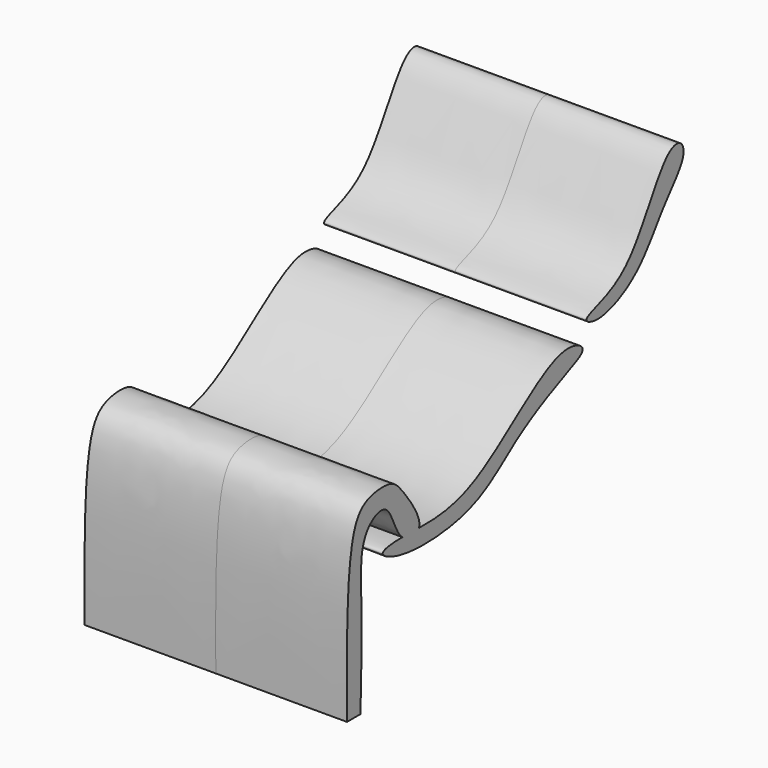
from build123d import *

# Parameters (mm, degrees)
F1_DEPTH = 63.5


with BuildPart() as f1:
    # F0 (on Right) → F1 (new body, symmetric)
    with BuildSketch(Plane.YZ):
        with BuildLine():
            add(Edge.make_bspline(
                [(-143.2403773069, -104.3510586023), (-142.7562305545, -88.6156108717), (-141.8814850282, -60.1848867372), (-144.5745803778, -27.8573641543), (-124.9688455585, -18.2280926487), (-122.6595201023, -35.2702398919), (-117.8873968399, -39.2565765031)],
                knots=[0, 0, 0, 0, 0.144009507, 0.260189796, 0.3348491633, 0.4268115335, 0.4268115335, 0.4268115335, 0.4268115335], degree=3))
            add(Edge.make_bspline(
                [(-117.8873968399, -39.2565765031), (-114.7446942469, -39.2553643323), (-111.3888290008, -39.3884462115), (-107.8556342883, -39.4389297117)],
                knots=[0, 0, 0, 0, 0.037982426, 0.037982426, 0.037982426, 0.037982426], degree=3))
            add(Edge.make_bspline(
                [(-107.8556342883, -39.4389297117), (-106.063178392, -35.3439779029), (-118.296132153, -18.3972227692), (-124.2406833684, -12.5728886668), (-138.4186777931, -13.1151114694), (-151.9247554576, -23.7874876821), (-151.6138692557, -70.8019272139), (-151.3920426369, -104.3510586023)],
                knots=[0.4939256363, 0.4939256363, 0.4939256363, 0.4939256363, 0.5938790041, 0.6592806539, 0.732580388, 0.809166244, 1, 1, 1, 1], degree=3))
            add(Edge.make_bspline(
                [(-151.3920426369, -104.3510586023), (-148.6748208602, -104.3510586023), (-145.9575990836, -104.3510586023), (-143.2403773069, -104.3510586023)],
                knots=[0, 0, 0, 0, 8.1516653299, 8.1516653299, 8.1516653299, 8.1516653299], degree=3))
        make_face()
        with BuildLine():
            add(Edge.make_bspline(
                [(-117.8873968399, -39.2565765031), (-114.4047030965, -42.165803447), (-109.0591862239, -42.1885020642), (-107.8556342883, -39.4389297117)],
                knots=[0.4268115335, 0.4268115335, 0.4268115335, 0.4268115335, 0.4939256363, 0.4939256363, 0.4939256363, 0.4939256363], degree=3))
            add(Edge.make_bspline(
                [(-107.8556342883, -39.4389297117), (-98.5103778433, -39.5724579472), (-69.6510901191, -38.3611280454), (-27.0967446465, 6.9957296893), (-3.7261879502, -3.5535051081), (-20.8971455397, -10.6520081189), (-49.7921916514, -24.3192169011), (-72.345637494, -47.096617427), (-117.0643868308, -49.4816010583), (-134.6082046549, -40.2850495858), (-124.0601600445, -39.2589573977), (-117.8873968399, -39.2565765031)],
                knots=[0.037982426, 0.037982426, 0.037982426, 0.037982426, 0.1384454745, 0.3118662471, 0.3895476597, 0.4628081726, 0.586770912, 0.7097739282, 0.8529230016, 0.925396529, 1, 1, 1, 1], degree=3))
        make_face()
        with BuildLine():
            add(Edge.make_bspline(
                [(-117.8873968399, -39.2565765031), (-114.7446942469, -39.2553643323), (-111.3888290008, -39.3884462115), (-107.8556342883, -39.4389297117)],
                knots=[0, 0, 0, 0, 0.037982426, 0.037982426, 0.037982426, 0.037982426], degree=3))
            add(Edge.make_bspline(
                [(-117.8873968399, -39.2565765031), (-114.4047030965, -42.165803447), (-109.0591862239, -42.1885020642), (-107.8556342883, -39.4389297117)],
                knots=[0.4268115335, 0.4268115335, 0.4268115335, 0.4268115335, 0.4939256363, 0.4939256363, 0.4939256363, 0.4939256363], degree=3))
        make_face()
    extrude(amount=F1_DEPTH, both=True)


with BuildPart() as f1b:
    # F0 (on Right) → F1, piece 2 (new body, symmetric)
    with BuildSketch(Plane.YZ):
        with BuildLine():
            add(Edge.make_bspline(
                [(0, 11.4993443713), (6.0327942829, 13.6499591816), (22.435885496, 19.9287356741), (39.4789125359, 60.6511323529), (51.3272792015, 61.5973777714), (53.8015059336, 52.1005124557), (38.3539545811, 36.7778983922), (25.8898720095, 13.8542040197), (1.9211276563, 3.3131087785), (-9.5565337921, 8.2085084616), (-3.4155903862, 10.2817296265), (0, 11.4993443713)],
                knots=[0, 0, 0, 0, 0.1307190982, 0.3074077359, 0.3820551266, 0.4517684437, 0.5748938362, 0.7180027825, 0.8540287658, 0.9259906978, 1, 1, 1, 1], degree=3))
        make_face()
    extrude(amount=F1_DEPTH, both=True)


solid = Compound([f1.part, f1b.part])
